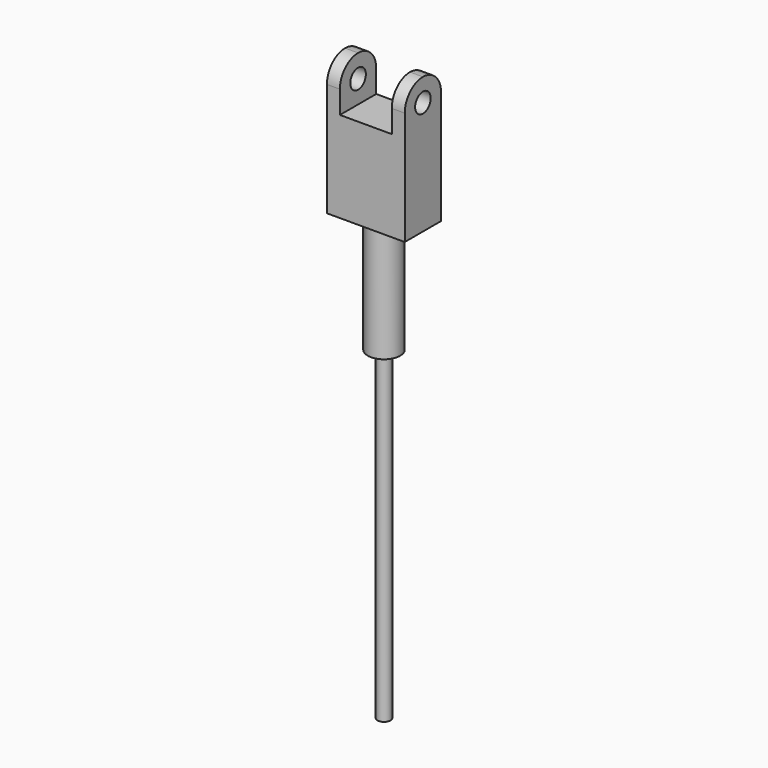
from build123d import *

# Parameters (mm, degrees)
F0_W      = 24
F0_H      = 14
F1_DEPTH  = 28
F2_W      = 4
F2_H      = 14
F3_DEPTH  = 14
F5_D      = 6
F6_R      = 6.99999
F7_R      = 5
F8_DEPTH  = 36
F9_R      = 2
F10_DEPTH = 100


# Not quite as in the source:
# - a fillet or chamfer is up to 0.001 mm smaller than in the source, because OpenCascade refuses the exact size


with BuildPart() as f1:
    # F0 (on Top) → F1 (new body)
    with BuildSketch(Plane.XY):
        with Locations((6.0259448364, -0.9606586885)):
            Rectangle(F0_W, F0_H)
    extrude(amount=-F1_DEPTH)

    # F2 (on face) → F3 (join)
    with BuildSketch(Plane.XY):
        with Locations((-3.9740551636, -0.9606586885)):
            Rectangle(F2_W, F2_H)
        with Locations((16.0259448364, -0.9606586885)):
            Rectangle(F2_W, F2_H)
    extrude(amount=F3_DEPTH)

    # F5 (through all)
    with Locations(Plane.YZ.offset(18.0259448364)):
        with Locations((-0.9606586885, 7)):
            Hole(F5_D / 2)

    # F6 (radius 7 in the source; OpenCascade refuses exactly that, so slightly less here)
    f6_edges = [f1.edges().sort_by_distance(p)[0] for p in [
        (16.025945, -7.960659, 14),
        (16.025945, 6.039341, 14),
        (-3.974055, 6.039341, 14),
        (-3.974055, -7.960659, 14),
    ]]
    fillet(f6_edges, radius=F6_R)

    # F7 (on face) → F8 (join)
    with BuildSketch(Plane(origin=(0, 0, -28), x_dir=(1, 0, 0), z_dir=(0, 0, -1))):
        with Locations((6.0259448364, 0.9606586885)):
            Circle(F7_R)
    extrude(amount=F8_DEPTH)

    # F9 (on face) → F10 (join)
    with BuildSketch(Plane(origin=(0, 0, -64), x_dir=(1, 0, 0), z_dir=(0, 0, -1))):
        with Locations((6.0259448364, 0.9606586885)):
            Circle(F9_R)
    extrude(amount=F10_DEPTH)


solid = f1.part
